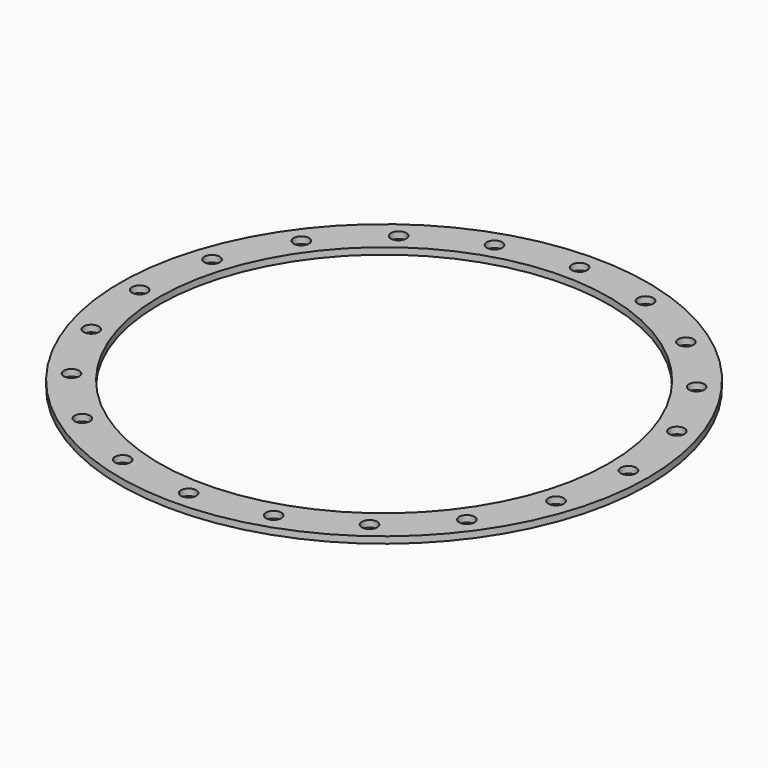
from build123d import *

# Parameters (mm, degrees)
F0_R     = 380.9121654934
F0_R_2   = 324.6612464713
F2_DEPTH = 9.525
F5_D     = 22.225


# Not quite as in the source:
# - a feature names something its author has since deleted; it is built from what else it names
# - the program builds the solid bodies; features that only make, move or delete a surface that nothing else refers to are left out


with BuildPart() as f2:
    # F0 (on Top) → F2 (new body)
    with BuildSketch(Plane.XY):
        Circle(F0_R)
        Circle(F0_R_2, mode=Mode.SUBTRACT)
    extrude(amount=F2_DEPTH)

    # F5 (through all)
    with Locations(Plane(origin=(0, 0, 0), x_dir=(1, 0, 0), z_dir=(0, 0, -1))):
        with Locations((-285.2887655833, -207.2744209584), (-335.3770581092, -108.9706118443), (-352.636307478, 0), (-335.3770581092, 108.9706118443), (-285.2887655833, 207.2744209584), (-207.2744209584, 285.2887655833), (-108.9706118443, 335.3770581092), (0, 352.636307478), (108.9706118443, 335.3770581092), (207.2744209584, 285.2887655833), (285.2887655833, 207.2744209584), (335.3770581092, 108.9706118443), (352.636307478, 0), (335.3770581092, -108.9706118443), (285.2887655833, -207.2744209584), (207.2744209584, -285.2887655833), (108.9706118443, -335.3770581092), (0, -352.636307478), (-108.9706118443, -335.3770581092), (-207.2744209584, -285.2887655833)):
            Hole(F5_D / 2)


solid = f2.part
